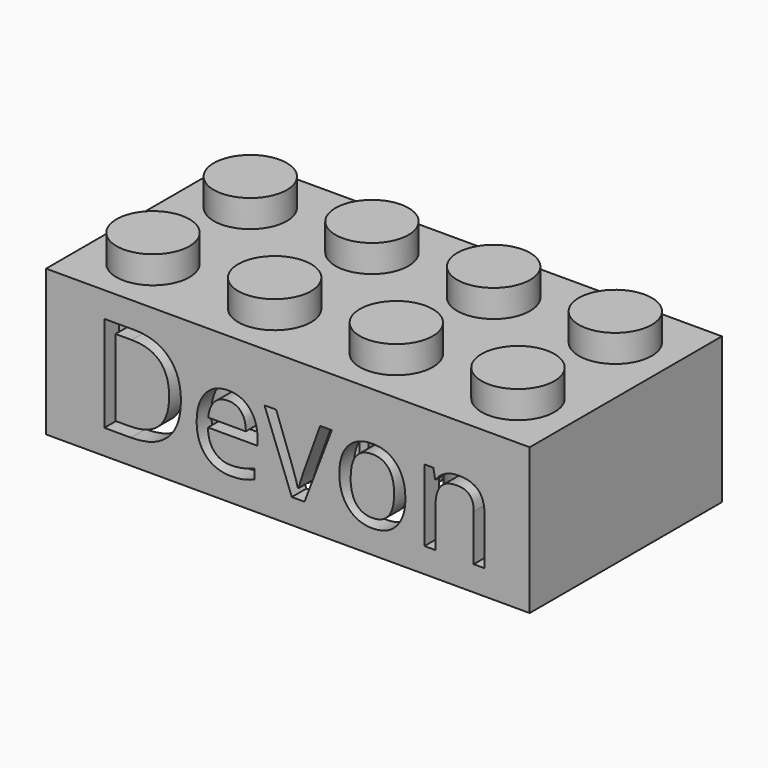
from build123d import *

# Parameters (mm, degrees)
F0_W          = 31.8
F0_H          = 15.8
F1_DEPTH      = 9.6
F2_W          = 29.4
F2_H          = 13.4
F3_DEPTH      = 8.4
F4_R          = 2.4
F5_DEPTH      = 1.8
F6_R          = 1.3
F7_DEPTH      = 1.2
F8_R          = 3.255
F8_R_2        = 2.4
F9_DEPTH      = 8.4
F10_W         = 0.6
F10_H         = 0.3
F11_DEPTH     = 8.4
F12_W         = 0.3
F12_H         = 0.6
F13_DEPTH     = 8.4
F14_W         = 0.8
F14_H         = 3.8
F15_DEPTH     = 6.4
F16_TEXT_SIZE = 8.8339524357
F17_DEPTH     = 1.2


# Not quite as in the source:
# - Text() gives the source's letters only with a copy of the font that has no kerning and outlines rounded to 1/6400 em; it was checked with that copy


with BuildPart() as f1:
    # F0 (on Top) → F1 (new body)
    with BuildSketch(Plane.XY):
        Rectangle(F0_W, F0_H)
    extrude(amount=F1_DEPTH)

    # F2 (on face) → F3 (cut)
    with BuildSketch(Plane(origin=(0, 0, 0), x_dir=(1, 0, 0), z_dir=(0, 0, -1))):
        Rectangle(F2_W, F2_H)
    extrude(amount=-F3_DEPTH, mode=Mode.SUBTRACT)

    # F4 (on face) → F5 (join)
    with BuildSketch(Plane.XY.offset(9.6)):
        with Locations((-11.95, 3.95)):
            Circle(F4_R)
        with Locations((-11.95, -4.05)):
            Circle(F4_R)
        with Locations((-3.95, 3.95)):
            Circle(F4_R)
        with Locations((-3.95, -4.05)):
            Circle(F4_R)
        with Locations((4.05, 3.95)):
            Circle(F4_R)
        with Locations((4.05, -4.05)):
            Circle(F4_R)
        with Locations((12.05, 3.95)):
            Circle(F4_R)
        with Locations((12.05, -4.05)):
            Circle(F4_R)
    extrude(amount=F5_DEPTH)

    # F6 (on face) → F7 (cut)
    with BuildSketch(Plane(origin=(0, 0, 8.4), x_dir=(1, 0, 0), z_dir=(0, 0, -1))):
        with Locations((-11.95, 3.95)):
            Circle(F6_R)
        with Locations((-11.95, -4.05)):
            Circle(F6_R)
        with Locations((-3.95, 3.95)):
            Circle(F6_R)
        with Locations((-3.95, -4.05)):
            Circle(F6_R)
        with Locations((4.05, 3.95)):
            Circle(F6_R)
        with Locations((4.05, -4.05)):
            Circle(F6_R)
        with Locations((12.05, 3.95)):
            Circle(F6_R)
        with Locations((12.05, -4.05)):
            Circle(F6_R)
    extrude(amount=-F7_DEPTH, mode=Mode.SUBTRACT)

    # F8 (on face) → F9 (join, through all)
    with BuildSketch(Plane(origin=(0, 0, 8.4), x_dir=(1, 0, 0), z_dir=(0, 0, -1))):
        with Locations((-7.95, -0.05)):
            Circle(F8_R)
        with Locations((-7.95, -0.05)):
            Circle(F8_R_2, mode=Mode.SUBTRACT)
        Circle(F8_R)
        Circle(F8_R_2, mode=Mode.SUBTRACT)
        with Locations((8.05, -0.05)):
            Circle(F8_R)
        with Locations((8.05, -0.05)):
            Circle(F8_R_2, mode=Mode.SUBTRACT)
    extrude(amount=F9_DEPTH)

    # F10 (on face) → F11 (join, through all)
    with BuildSketch(Plane(origin=(0, 0, 0), x_dir=(1, 0, 0), z_dir=(0, 0, -1))):
        with Locations((-11.95, 6.55)):
            Rectangle(F10_W, F10_H)
        with Locations((-11.95, -6.55)):
            Rectangle(F10_W, F10_H)
        with Locations((-3.95, 6.55)):
            Rectangle(F10_W, F10_H)
        with Locations((-3.95, -6.55)):
            Rectangle(F10_W, F10_H)
        with Locations((4.05, 6.55)):
            Rectangle(F10_W, F10_H)
        with Locations((4.05, -6.55)):
            Rectangle(F10_W, F10_H)
        with Locations((12.05, 6.55)):
            Rectangle(F10_W, F10_H)
        with Locations((12.05, -6.55)):
            Rectangle(F10_W, F10_H)
    extrude(amount=-F11_DEPTH)

    # F12 (on face) → F13 (join, through all)
    with BuildSketch(Plane(origin=(0, 0, 0), x_dir=(1, 0, 0), z_dir=(0, 0, -1))):
        with Locations((-14.55, 4.05)):
            Rectangle(F12_W, F12_H)
        with Locations((-14.55, -3.95)):
            Rectangle(F12_W, F12_H)
        with Locations((14.55, 4.05)):
            Rectangle(F12_W, F12_H)
        with Locations((14.55, -3.95)):
            Rectangle(F12_W, F12_H)
    extrude(amount=-F13_DEPTH)

    # F14 (on face) → F15 (join)
    with BuildSketch(Plane(origin=(0, 0, 8.4), x_dir=(1, 0, 0), z_dir=(0, 0, -1))):
        with Locations((0, 5)):
            Rectangle(F14_W, F14_H)
        with Locations((0, -5)):
            Rectangle(F14_W, F14_H)
    extrude(amount=F15_DEPTH)

    # F16 (on face) → F17 (cut)
    with BuildSketch(Plane.XZ.offset(7.9)):
        with Locations((-12.9348387929, 1.6303084558)):
            Text('Devon', F16_TEXT_SIZE, font='Open Sans', text_align=(TextAlign.LEFT, TextAlign.BOTTOM))
    extrude(amount=-F17_DEPTH, mode=Mode.SUBTRACT)


solid = f1.part
